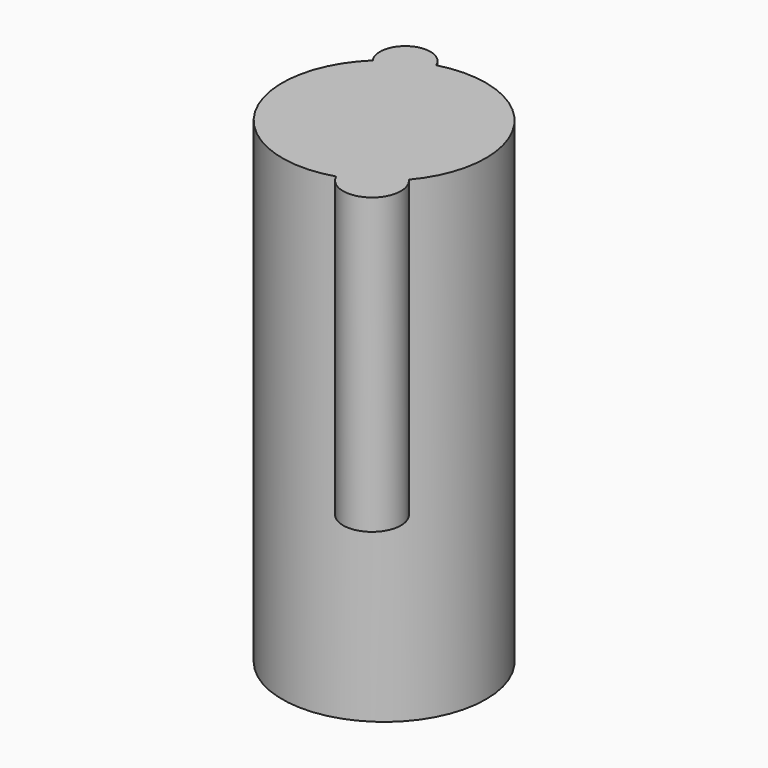
from build123d import *

# Parameters (mm, degrees)
F1_R     = 21.7223344902
F2_DEPTH = 101.6
F4_DEPTH = 99.02421
F3_R     = 6.1579906
F3_R_2   = 5.385299851
F5_DEPTH = 62.76523


# Not quite as in the source:
# - a feature names something its author has since deleted; it is built from what else it names


with BuildPart() as f2:
    # F1 (on Top) → F2 (new body)
    with BuildSketch(Plane.XY):
        Circle(F1_R)
    extrude(amount=F2_DEPTH)

    # F3 (on face) → F4 (join)
    with BuildSketch(Plane.XY.offset(101.6)):
        with BuildLine():
            ThreePointArc((6.3684736853, -20.7678202666), (11.9405298036, -18.1461721505), (16.5529894413, -14.0662132879))
            ThreePointArc((16.5529894413, -14.0662132879), (8.5555496891, -13.0019756287), (6.3684736853, -20.7678202666))
        make_face()
    extrude(amount=-F4_DEPTH)

    # F3 (on face) → F5 (join)
    with BuildSketch(Plane.XY.offset(101.6)):
        with Locations((11.9405298036, -18.1461721505)):
            Circle(F3_R)
        with Locations((-10.6482523042, 18.933423847)):
            Circle(F3_R_2)
    extrude(amount=-F5_DEPTH)


solid = f2.part
